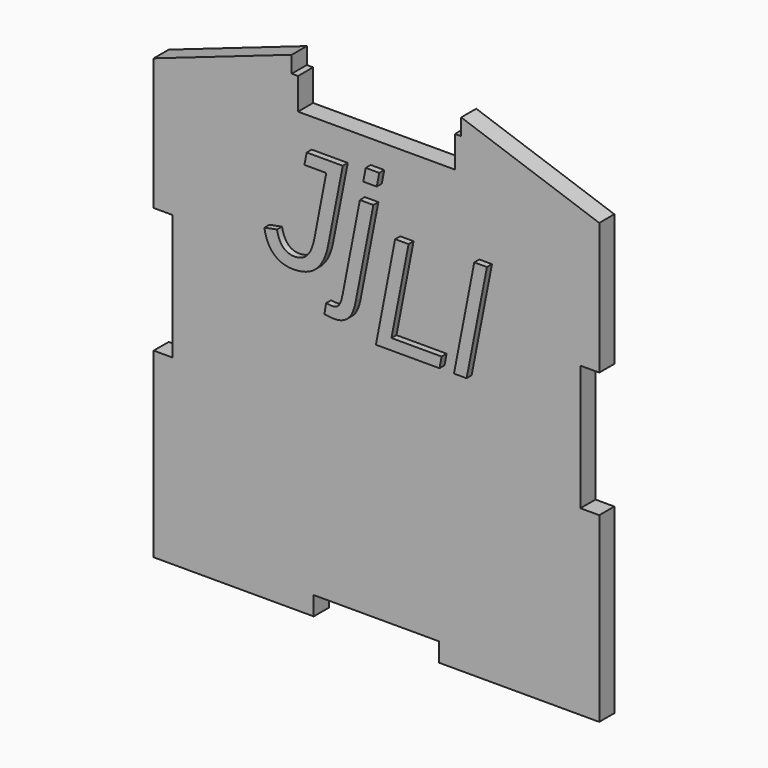
from build123d import *

# Parameters (mm, degrees)
F1_DEPTH       = 3
F2_TEXT_SIZE   = 24.4788678524
F2_TEXT_SIZE_2 = 22.9843778057
F3_DEPTH       = 1


# Not quite as in the source:
# - Text() gives the source's letters only with a copy of the font that has no kerning and outlines rounded to 1/6400 em; it was checked with that copy


with BuildPart() as f1:
    # F0 (on Front) → F1 (new body)
    with BuildSketch(Plane.XZ):
        Polygon((-12.5, 31), (-35.5, 31), (-35.5, 10), (-32.5, 10), (-32.5, -10), (-35.5, -10), (-35.5, -39), (-10, -39), (-10, -36), (10, -36), (10, -39), (35.5, -39), (35.5, -10), (32.5, -10), (32.5, 10), (35.5, 10), (35.5, 31), (12.5, 31), align=None)
        Polygon((-13.5, 38.652173913), (-35.5, 31), (-12.5, 31), (-12.5, 36), (-13.5, 36), align=None)
        Polygon((12.5, 36), (12.5, 31), (35.5, 31), (13.5, 38.652173913), (13.5, 36), align=None)
    extrude(amount=F1_DEPTH)

    # F2 (on face) → F3 (join)
    with BuildSketch(Plane.XZ.offset(3)):
        with Locations((-17, 9.5487520201)):
            Text('Jj', F2_TEXT_SIZE, font='Arimo', font_style=FontStyle.ITALIC, text_align=(TextAlign.LEFT, TextAlign.BOTTOM))
        with Locations((0, 3)):
            Text('Ll', F2_TEXT_SIZE_2, font='Arimo', font_style=FontStyle.ITALIC, text_align=(TextAlign.LEFT, TextAlign.BOTTOM))
    extrude(amount=F3_DEPTH)


solid = f1.part
